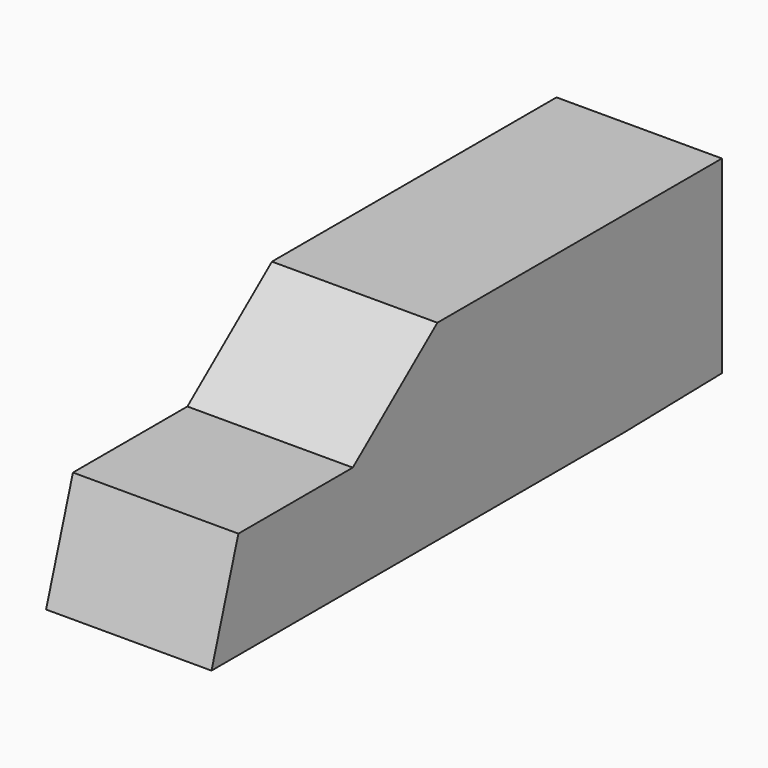
from build123d import *

# Parameters (mm, degrees)
F1_DEPTH = 25.4


# Not quite as in the source:
# - a feature names something its author has since deleted; it is built from what else it names


with BuildPart() as f1:
    # F0 (on Right) → F1 (new body)
    with BuildSketch(Plane.YZ):
        Polygon((-16.2311457098, 0), (-38.1909310818, 0), (-43.3467067778, -16.4221003652), (35.8994752169, -16.4221003652), (54.6130314469, -16.0401910543), (54.6130314469, 12.9849165678), (35.8994752169, 12.9849165678), (0, 12.9849165678), align=None)
    extrude(amount=F1_DEPTH)


solid = f1.part
